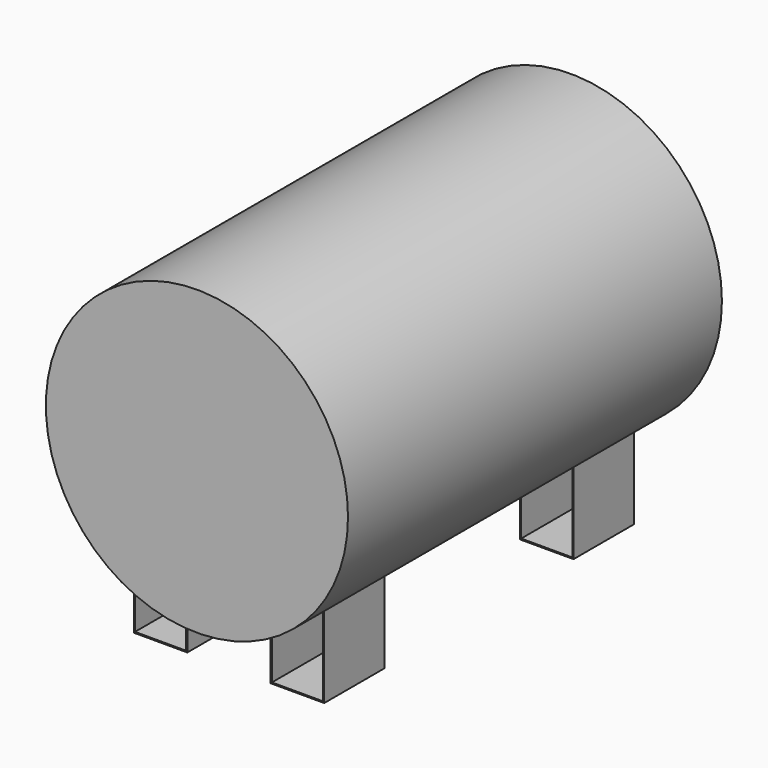
from build123d import *

# Parameters (mm, degrees)
F0_R     = 609.6
F1_DEPTH = 1873.25
F4_DEPTH = 304.8


# Not quite as in the source:
# - a feature of the source that left no trace in its solid (it failed there, or was rolled back) is left out
# - a pattern or mirror of a feature is missing from the dataset's text; its kind, count and spacing are read off the source's solid


with BuildPart() as f1:
    # F0 (on Front) → F1 (new body)
    with BuildSketch(Plane.XZ):
        Circle(F0_R)
    extrude(amount=-F1_DEPTH)

    # F1_copies: F1 across plane


with BuildPart() as f1_1:
    add(f1.part)
    add(f1.part.mirror(Plane(origin=(0, 930.275, 0), x_dir=(0, 0, -1), z_dir=(0, -1, 0))))

    # F3 (on offset) → F4 (join)
    with BuildSketch(Plane.XZ.offset(-149.225)):
        with BuildLine():
            Line((-384.175, -473.3093379334), (-384.175, -800.1))
            Line((-384.175, -800.1), (-168.275, -800.1))
            Line((-168.275, -800.1), (-168.275, -585.9144002113))
            ThreePointArc((-168.275, -585.9144002113), (-170.6576627394, -585.2248475145), (-173.0375, -584.5256055929))
            Line((-173.0375, -584.5256055929), (-173.0375, -795.3375))
            Line((-173.0375, -795.3375), (-379.4125, -795.3375))
            Line((-379.4125, -795.3375), (-379.4125, -477.1355308964))
            ThreePointArc((-379.4125, -477.1355308964), (-381.7985430528, -475.2284003748), (-384.175, -473.3093379334))
        make_face()
    f4 = extrude(amount=-F4_DEPTH)

    # F4_copies: F4 across plane
    add(f4.mirror(Plane.ZX.offset(930.275)))

    # F5: F1 across plane


with BuildPart() as f1_2:
    add(f1_1.part)
    add(f1_1.part.mirror(Plane.YZ))


solid = f1_2.part
